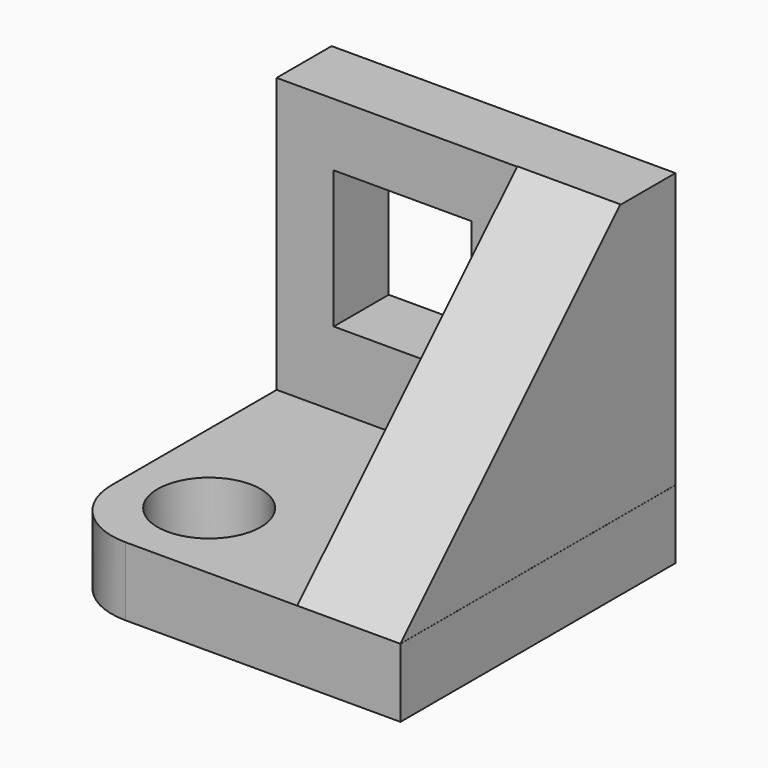
from build123d import *

# Parameters (mm, degrees)
F0_W      = 100
F0_H      = 100
F1_DEPTH  = 20
F2_W      = 100
F2_H      = 80
F3_DEPTH  = 20
F4_W      = 30
F4_H      = 80
F5_DEPTH  = 80
F6_R      = 20
F7_R      = 15
F8_DEPTH  = 20
F9_W      = 40
F9_H      = 40
F10_DEPTH = 20
F11_SIZE  = 79.99999


# Not quite as in the source:
# - a fillet or chamfer is up to 0.001 mm smaller than in the source, because OpenCascade refuses the exact size


with BuildPart() as f1:
    # F0 (on Top) → F1 (new body)
    with BuildSketch(Plane.XY):
        with Locations((0.1719114778, -50)):
            Rectangle(F0_W, F0_H)
    extrude(amount=F1_DEPTH)

    # F2 (on Front) → F3 (join)
    with BuildSketch(Plane.XZ):
        with Locations((0.1466497779, 59.8839402659)):
            Rectangle(F2_W, F2_H)
    extrude(amount=F3_DEPTH)

    # F4 (on face) → F5 (join)
    with BuildSketch(Plane.XY.offset(20)):
        with Locations((35.1466497779, -60)):
            Rectangle(F4_W, F4_H)
    extrude(amount=F5_DEPTH)

    # F6
    f6_edges = [f1.edges().sort_by_distance(p)[0] for p in [
        (-49.828089, -100, 10),
    ]]
    fillet(f6_edges, radius=F6_R)

    # F7 (on face) → F8 (cut)
    with BuildSketch(Plane.XY.offset(20)):
        with Locations((-25.480100885, -75)):
            Circle(F7_R)
    extrude(amount=-F8_DEPTH, mode=Mode.SUBTRACT)

    # F9 (on face) → F10 (cut)
    with BuildSketch(Plane.XZ.offset(20)):
        with Locations((-13.2386269793, 61.6098302603)):
            Rectangle(F9_W, F9_H)
    extrude(amount=-F10_DEPTH, mode=Mode.SUBTRACT)

    # F11 (size 80 in the source; OpenCascade refuses exactly that, so slightly less here)
    f11_edges = [f1.edges().sort_by_distance(p)[0] for p in [
        (35.14665, -100, 100),
    ]]
    chamfer(f11_edges, length=F11_SIZE)


solid = f1.part
